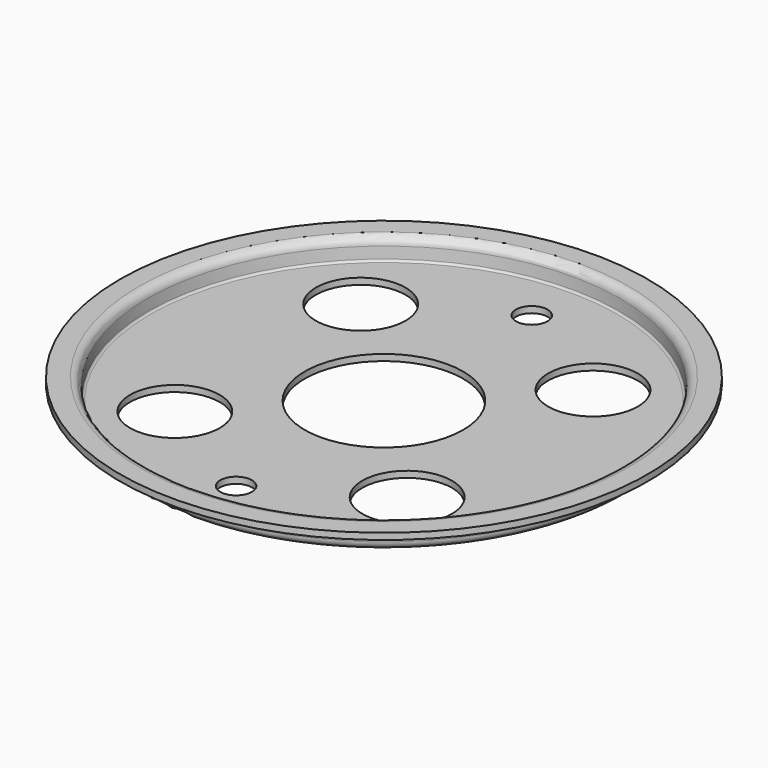
from build123d import *

# Parameters (mm, degrees)
F2_R     = 42.5
F2_R_2   = 75
F2_R_3   = 15
F3_DEPTH = 25


# Not quite as in the source:
# - ends of sketch curves that miss each other by under 0.0002 mm in the source are joined


with BuildPart() as f1:
    # F0 (on Front) → F1 (revolve)
    with BuildSketch(Plane.XZ):
        with BuildLine():
            Line((-221.3601278806, 0), (0, 0))
            Line((0, 0), (0, 6))
            Line((0, 6), (-221.3601278806, 6))
            ThreePointArc((-221.3601278806, 6), (-222.7368362926, 6.5492520372), (-223.3573858774, 7.8953281437))
            Line((-223.3573858774, 7.8953281437), (-223.9088928554, 18.4186876499))
            ThreePointArc((-223.9088928554, 18.4186876499), (-226.3910925279, 23.8029949681), (-231.8979291334, 26))
            Line((-231.8979291334, 26), (-250, 26))
            Line((-250, 26), (-250, 20))
            Line((-250, 20), (-231.8979291334, 20))
            ThreePointArc((-231.8979291334, 20), (-230.521219982, 19.450748742), (-229.9006700639, 18.1046719125))
            Line((-229.9006700639, 18.1046719125), (-229.3491641587, 7.5813123501))
            ThreePointArc((-229.3491641587, 7.5813123501), (-226.8669644862, 2.1970050319), (-221.3601278806, 0))
        make_face()
    revolve(axis=Axis((0, 0, 34.008089453), (0, 0, 1)))

    # F2 (on Top) → F3 (cut)
    with BuildSketch(Plane.XY):
        with Locations((-110, -110)):
            Circle(F2_R)
        with Locations((110, -110)):
            Circle(F2_R)
        with Locations((110, 110)):
            Circle(F2_R)
        with Locations((-110, 110)):
            Circle(F2_R)
        Circle(F2_R_2)
        with Locations((0, -175)):
            Circle(F2_R_3)
        with Locations((0, 175)):
            Circle(F2_R_3)
    extrude(amount=F3_DEPTH, mode=Mode.SUBTRACT)


solid = f1.part
